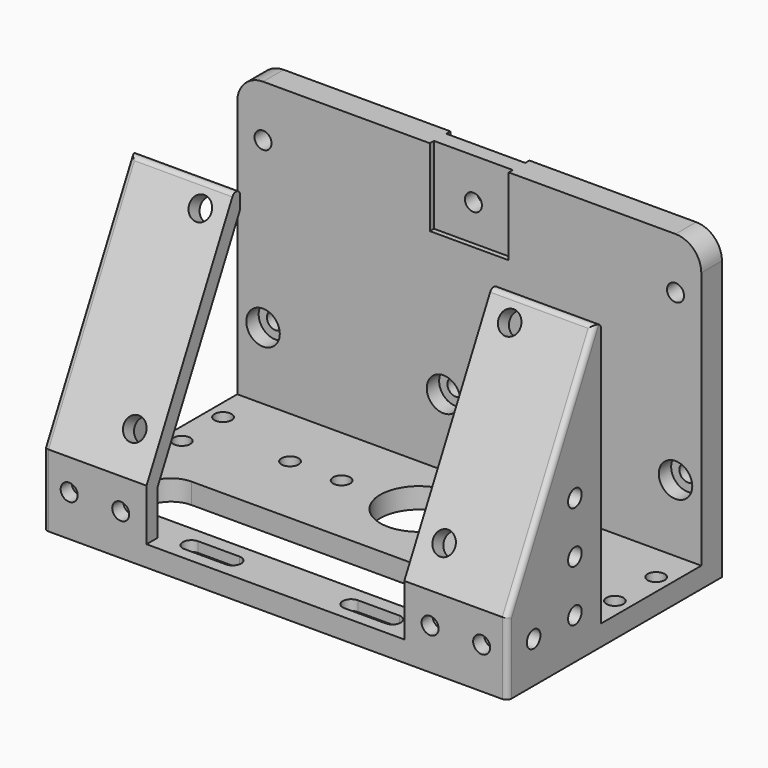
from build123d import *

# Parameters (mm, degrees)
F0_W      = 90
F0_H      = 52
F0_R      = 1.65
F0_R_2    = 7.5
F0_W_2    = 2.5
F0_H_2    = 10
F1_DEPTH  = 4
F2_DEPTH  = 3
F3_W      = 90
F3_H      = 5
F4_DEPTH  = 55
F5_W      = 15.3
F5_H      = 1
F6_DEPTH  = 15
F7_R      = 1.65
F8_DEPTH  = 3
F9_R      = 1.65
F10_DEPTH = 5
F11_R     = 3.25
F12_DEPTH = 3
F14_DEPTH = 2
F16_DEPTH = 3
F17_DEPTH = 20
F18_R     = 2.15
F19_DEPTH = 3
F20_R     = 1.65
F21_DEPTH = 2.6730195726
F22_R     = 1.65
F23_DEPTH = 3
F24_R     = 1
F25_R     = 5


# Not quite as in the source:
# - a pattern or mirror of a feature is missing from the dataset's text; its kind, count and spacing are read off the source's solid
# - a feature names something its author has since deleted; it is built from what else it names


with BuildPart() as f1:
    # F0 (on Top) → F1 (new body)
    with BuildSketch(Plane.XY):
        with Locations((0, -8.8)):
            Rectangle(F0_W, F0_H)
        with BuildLine():
            ThreePointArc((-19.5, -32.45), (-21.15, -30.8), (-19.5, -29.15))
            Line((-19.5, -29.15), (-11.5, -29.15))
            ThreePointArc((-11.5, -29.15), (-10.333273811, -29.633273811), (-9.85, -30.8))
            ThreePointArc((-9.85, -30.8), (-10.333273811, -31.966726189), (-11.5, -32.45))
            Line((-11.5, -32.45), (-19.5, -32.45))
        make_face(mode=Mode.SUBTRACT)
        with BuildLine():
            ThreePointArc((19.5, -29.15), (20.666726189, -29.633273811), (21.15, -30.8))
            ThreePointArc((21.15, -30.8), (20.666726189, -31.966726189), (19.5, -32.45))
            Line((19.5, -32.45), (11.5, -32.45))
            ThreePointArc((11.5, -32.45), (9.85, -30.8), (11.5, -29.15))
            Line((11.5, -29.15), (19.5, -29.15))
        make_face(mode=Mode.SUBTRACT)
        Polygon((-35, -2), (-35, -12), (35, -12), (35, -2), (37.5, -2), (37.5, -12), (37.5, -14.5), (37.5, -26.5), (-37.5, -26.5), (-37.5, -14.5), (-37.5, -12), (-37.5, -2), align=None, mode=Mode.SUBTRACT)
        with Locations((-42, -5)):
            Circle(F0_R, mode=Mode.SUBTRACT)
        with Locations((-25, 0)):
            Circle(F0_R, mode=Mode.SUBTRACT)
        with Locations((-15, 0)):
            Circle(F0_R, mode=Mode.SUBTRACT)
        with Locations((-42, 5)):
            Circle(F0_R, mode=Mode.SUBTRACT)
        Circle(F0_R_2, mode=Mode.SUBTRACT)
        with Locations((15, 0)):
            Circle(F0_R, mode=Mode.SUBTRACT)
        with Locations((42, -5)):
            Circle(F0_R, mode=Mode.SUBTRACT)
        with Locations((25, 0)):
            Circle(F0_R, mode=Mode.SUBTRACT)
        with Locations((42, 5)):
            Circle(F0_R, mode=Mode.SUBTRACT)
        Polygon((35, -12), (-35, -12), (-37.5, -12), (-37.5, -14.5), (37.5, -14.5), (37.5, -12), align=None)
        with Locations((-36.25, -7)):
            Rectangle(F0_W_2, F0_H_2)
        with Locations((36.25, -7)):
            Rectangle(F0_W_2, F0_H_2)
    extrude(amount=F1_DEPTH)

    # F0 (on Top) → F2 (join)
    with BuildSketch(Plane.XY):
        with Locations((-36.25, -7)):
            Rectangle(F0_W_2, F0_H_2)
        with Locations((36.25, -7)):
            Rectangle(F0_W_2, F0_H_2)
    extrude(amount=F2_DEPTH)

    # F3 (on face) → F4 (join)
    with BuildSketch(Plane.XY.offset(4)):
        with Locations((0, 14.7)):
            Rectangle(F3_W, F3_H)
    extrude(amount=F4_DEPTH)

    # F5 (on face) → F6 (cut)
    with BuildSketch(Plane.XY.offset(59)):
        with Locations((0, 16.7)):
            Rectangle(F5_W, F5_H)
        with Locations((0, 12.7)):
            Rectangle(F5_W, F5_H)
    extrude(amount=-F6_DEPTH, mode=Mode.SUBTRACT)

    # F7 (on face) → F8 (cut, through all)
    with BuildSketch(Plane(origin=(0, 16.2, 0), x_dir=(-1, 0, 0), z_dir=(0, 1, 0))):
        with Locations((0, 51)):
            Circle(F7_R)
    extrude(amount=-F8_DEPTH, mode=Mode.SUBTRACT)

    # F9 (on face) → F10 (cut, through all)
    with BuildSketch(Plane(origin=(0, 17.2, 0), x_dir=(-1, 0, 0), z_dir=(0, 1, 0))):
        with Locations((-40, 17)):
            Circle(F9_R)
        with Locations((-5, 17)):
            Circle(F9_R)
        with Locations((40, 17)):
            Circle(F9_R)
        with Locations((5, 17)):
            Circle(F9_R)
        with Locations((-40, 49)):
            Circle(F9_R)
        with Locations((40, 49)):
            Circle(F9_R)
    extrude(amount=-F10_DEPTH, mode=Mode.SUBTRACT)

    # F11 (on face) → F12 (cut)
    with BuildSketch(Plane.XZ.offset(-12.2)):
        with Locations((5, 17)):
            Circle(F11_R)
        with Locations((40, 17)):
            Circle(F11_R)
        with Locations((-5, 17)):
            Circle(F11_R)
        with Locations((-40, 17)):
            Circle(F11_R)
    extrude(amount=-F12_DEPTH, mode=Mode.SUBTRACT)

    # F13 (on face) → F14 (cut)
    with BuildSketch(Plane.XY):
        with BuildLine():
            ThreePointArc((-22.5, -30.8), (-21.6213203436, -32.9213203436), (-19.5, -33.8))
            Line((-19.5, -33.8), (-11.5, -33.8))
            ThreePointArc((-11.5, -33.8), (-9.3786796564, -32.9213203436), (-8.5, -30.8))
            ThreePointArc((-8.5, -30.8), (-9.3786796564, -28.6786796564), (-11.5, -27.8))
            Line((-11.5, -27.8), (-19.5, -27.8))
            ThreePointArc((-19.5, -27.8), (-21.6213203436, -28.6786796564), (-22.5, -30.8))
        make_face()
        with BuildLine():
            Line((-11.5, -32.45), (-19.5, -32.45))
            ThreePointArc((-19.5, -32.45), (-21.15, -30.8), (-19.5, -29.15))
            Line((-19.5, -29.15), (-11.5, -29.15))
            ThreePointArc((-11.5, -29.15), (-10.333273811, -29.633273811), (-9.85, -30.8))
            ThreePointArc((-9.85, -30.8), (-10.333273811, -31.966726189), (-11.5, -32.45))
        make_face(mode=Mode.SUBTRACT)
        with BuildLine():
            ThreePointArc((8.5, -30.8), (9.3786796564, -32.9213203436), (11.5, -33.8))
            Line((11.5, -33.8), (19.5, -33.8))
            ThreePointArc((19.5, -33.8), (21.6213203436, -32.9213203436), (22.5, -30.8))
            ThreePointArc((22.5, -30.8), (21.6213203436, -28.6786796564), (19.5, -27.8))
            Line((19.5, -27.8), (11.5, -27.8))
            ThreePointArc((11.5, -27.8), (9.3786796564, -28.6786796564), (8.5, -30.8))
        make_face()
        with BuildLine():
            Line((11.5, -29.15), (19.5, -29.15))
            ThreePointArc((19.5, -29.15), (20.666726189, -29.633273811), (21.15, -30.8))
            ThreePointArc((21.15, -30.8), (20.666726189, -31.966726189), (19.5, -32.45))
            Line((19.5, -32.45), (11.5, -32.45))
            ThreePointArc((11.5, -32.45), (9.85, -30.8), (11.5, -29.15))
        make_face(mode=Mode.SUBTRACT)
    extrude(amount=F14_DEPTH, mode=Mode.SUBTRACT)

    # F15 (on face) → F16 (join)
    with BuildSketch(Plane.YZ.offset(45)):
        Polygon((-34.8, 14), (-34.8, 4), (-32.1269804274, 4), (-32.1269804274, 12.6380285008), align=None)
        Polygon((-12.100475013, 58.5503262094), (-34.8, 14), (-32.1269804274, 12.6380285008), (-12.100475013, 51.9422584157), align=None)
        Polygon((-32.1269804274, 12.6380285008), (-32.1269804274, 4), (-12.100475013, 4), (-12.100475013, 51.9422584157), align=None)
    f16 = extrude(amount=-F16_DEPTH)

    # F16_copies: F16 across plane
    add(f16.mirror(Plane(origin=(0, 0, 0), x_dir=(0, 0, -1), z_dir=(-1, 0, 0))))

    # F15 (on face) → F17 (join)
    with BuildSketch(Plane.YZ.offset(45)):
        Polygon((-34.8, 14), (-34.8, 4), (-32.1269804274, 4), (-32.1269804274, 12.6380285008), align=None)
        Polygon((-12.100475013, 58.5503262094), (-34.8, 14), (-32.1269804274, 12.6380285008), (-12.100475013, 51.9422584157), align=None)
    f17 = extrude(amount=-F17_DEPTH)

    # F17_copies: F17 across plane
    add(f17.mirror(Plane(origin=(0, 0, 0), x_dir=(0, 0, -1), z_dir=(-1, 0, 0))))

    # F18 (on face) → F19 (cut, through all)
    with BuildSketch(Plane(origin=(0, -33.2905823505, 16.9623989361), x_dir=(1, 0, 0), z_dir=(0, -0.8910065242, 0.4539904997))):
        with Locations((30, 4.1752219477)):
            Circle(F18_R)
        with Locations((30, 39.1752219477)):
            Circle(F18_R)
    f19 = extrude(amount=-F19_DEPTH, mode=Mode.SUBTRACT)

    # F19_copies: F19 across plane
    add(f19.mirror(Plane(origin=(0, 0, 0), x_dir=(0, 0, -1), z_dir=(-1, 0, 0))), mode=Mode.SUBTRACT)

    # F20 (on face) → F21 (cut, through all)
    with BuildSketch(Plane.XZ.offset(34.8)):
        with Locations((40, 8)):
            Circle(F20_R)
        with Locations((30, 8)):
            Circle(F20_R)
    f21 = extrude(amount=-F21_DEPTH, mode=Mode.SUBTRACT)

    # F21_copies: F21 across plane
    add(f21.mirror(Plane(origin=(0, 0, 0), x_dir=(0, 0, -1), z_dir=(-1, 0, 0))), mode=Mode.SUBTRACT)

    # F22 (on face) → F23 (cut, through all)
    with BuildSketch(Plane.YZ.offset(45)):
        with Locations((-28.4502375065, 8)):
            Circle(F22_R)
        with Locations((-18.4502375065, 8)):
            Circle(F22_R)
        with Locations((-18.4502375065, 18)):
            Circle(F22_R)
        with Locations((-18.4502375065, 28)):
            Circle(F22_R)
    f23 = extrude(amount=-F23_DEPTH, mode=Mode.SUBTRACT)

    # F23_copies: F23 across plane
    add(f23.mirror(Plane(origin=(0, 0, 0), x_dir=(0, 0, -1), z_dir=(-1, 0, 0))), mode=Mode.SUBTRACT)

    # F24
    f24_edges = [f1.edges().sort_by_distance(p)[0] for p in [
        (35, -12.100475, 58.550326),
        (45, -34.8, 7),
        (45, -23.450238, 36.275163),
        (-45, -34.8, 7),
        (-45, -23.450238, 36.275163),
        (-35, -12.100475, 58.550326),
    ]]
    fillet(f24_edges, radius=F24_R)

    # F25
    f25_edges = [f1.edges().sort_by_distance(p)[0] for p in [
        (45, 14.7, 59),
        (-45, 14.7, 59),
        (37.5, -26.5, 2),
        (37.5, -14.5, 2),
        (-37.5, -14.5, 2),
        (-37.5, -26.5, 2),
    ]]
    fillet(f25_edges, radius=F25_R)


solid = f1.part
